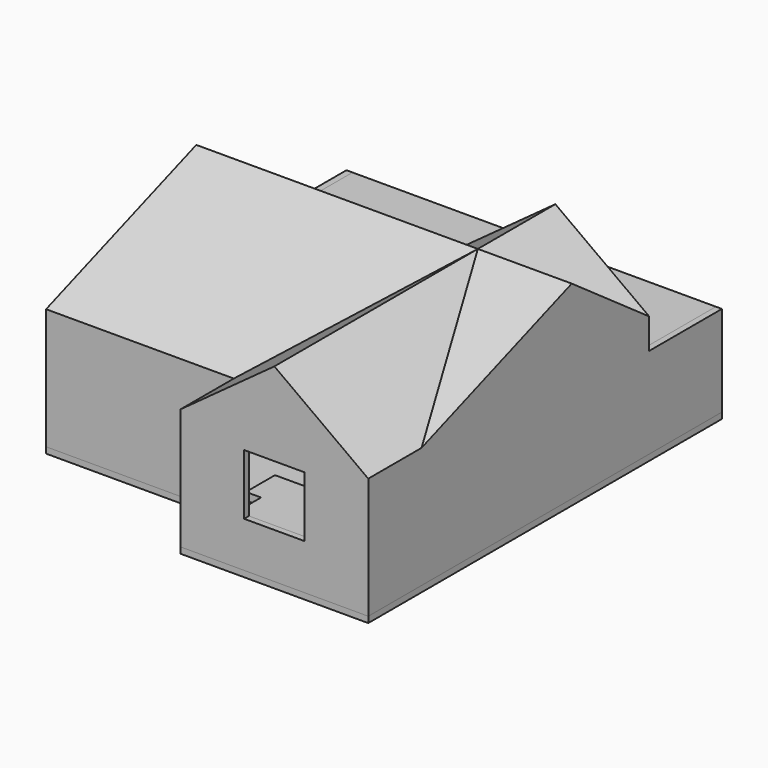
from build123d import *

# Parameters (mm, degrees)
F14_DEPTH    = 12400
F15_W        = 2000
F15_H        = 1000
F0_DEPTH     = 11600
F16_DEPTH    = 4000
F1_T         = 200
F1_T3_DEPTH  = 7689.8774544047
F1_T5_DEPTH  = 5394.2279984236
F1_T7_DEPTH  = 5394.2279984236
F1_T9_DEPTH  = 7689.8774544047
F1_T11_DEPTH = 4400
F2_W         = 2000
F2_H         = 2000
F17_DEPTH    = 2400
F18_DEPTH    = 200
F3_W         = 1000
F3_H         = 500
F3_W_2       = 500
F3_H_2       = 1000
F3_H_3       = 200
F4_DEPTH     = 200
F5_START     = -2800
F5_DEPTH     = 200
F6_START     = -1200
F6_DEPTH     = 300
F7_START     = -1450
F7_DEPTH     = 300
F19_START    = -1700
F19_DEPTH    = 300
F20_START    = -1950
F20_DEPTH    = 300
F21_START    = -2200
F21_DEPTH    = 300
F8_START     = -2450
F8_DEPTH     = 300
F22_START    = -2700
F22_DEPTH    = 300
F9_START     = -950
F9_DEPTH     = 300
F10_START    = -700
F10_DEPTH    = 300
F11_START    = -450
F11_DEPTH    = 300
F23_START    = -200
F23_DEPTH    = 300
F12_DEPTH    = 250


# Not quite as in the source:
# - an extrude ends at something that could not be found from the text; its depth is read off the source's solid
# - a shell that OpenCascade refuses in one call is made with other operations: the cavity is built on its own and cut out


with BuildPart() as f14:
    # F13 (on Right) → F14 (new body)
    with BuildSketch(Plane.YZ):
        Polygon((-6200, 0), (6200, 0), (6200, 3000), (3200, 3000), (3200, 4000), (0, 6256.6154524505), (-6200, 4000), align=None)
    extrude(amount=F14_DEPTH)

    # F15 (on face) → F0 (join)
    with BuildSketch(Plane(origin=(0, 3200, 0), x_dir=(-1, 0, 0), z_dir=(0, 1, 0))):
        Polygon((-9300, 6256.6154524505), (-12400, 4000), (-10300, 4000), (-10300, 5000), (-8300, 5000), (-8300, 4000), (-6200, 4000), align=None)
        with Locations((-9300, 4500)):
            Rectangle(F15_W, F15_H)
    extrude(amount=-F0_DEPTH)

    # F16 (add, through all): a face of the model
    f16_faces = [f14.faces().sort_by_distance(p)[0] for p in [
        (9300, -7300, 4000),
    ]]
    extrude(f16_faces, amount=F16_DEPTH)

    # F1: shell of thickness 200, made by hand


with BuildPart() as f1_core1:
    # F1_t2: copy of F14
    add(f14.part)

    # the walls: a layer under each face that stays
    f1_faces = [f1_core1.faces().sort_by_distance(p)[0] for p in [
        (4650, -3100, 5128.3077262252),
        (4650, 1600, 5128.3077262252),
        (10333.3333333333, 3200, 3542.7692420751),
        (9816.6666666667, 1600, 5880.512877042),
        (11883.3333333333, 1600, 5128.3077262252),
        (11883.3333333333, -1033.3333333333, 5880.512877042),
        (10850, -4200, 5128.3077262252),
        (9300, -8400, 3128.3077262252),
        (6200, -7300, 2000),
        (12400, -1100, 3128.3077262252),
        (7750, 2666.6666666667, 5128.3077262252),
        (7750, -4200, 5128.3077262252),
        (3100, -6200, 2000),
        (0, 0, 3128.3077262252),
    ]]
    thicken(f1_faces, amount=-F1_T, mode=Mode.SUBTRACT)

    # F1_s4 → F1_t3 (cut)
    with BuildSketch(Plane(origin=(-679.6785869535, -1359.357173907, -494.7655490384), x_dir=(-0.894427191, 0.4472135955, 0), z_dir=(0.4252472033, 0.8504944066, 0.3095546484))):
        Polygon((-8317.4260033625, 4665.513258174), (-8287.5816646932, 4464.1897106586), (-8360.6155438547, 4452.8857222652), (-8423.4513815758, 4491.7879735735), align=None)
    extrude(amount=F1_T3_DEPTH, mode=Mode.SUBTRACT)

    # F1_s6 → F1_t5 (cut)
    with BuildSketch(Plane(origin=(5462.1086087811, -5638.3056606773, 3976.089899851), x_dir=(-0.7182402228, -0.6957952158, 0), z_dir=(-0.6207165554, 0.6407396701, -0.4518447002))):
        Polygon((-6679.5906506398, 2661.3103147543), (-6599.4357743978, 2474.4492579485), (-6682.2486847174, 2438.2000137734), (-6764.1744994282, 2476.4118797687), align=None)
    extrude(amount=F1_T5_DEPTH, mode=Mode.SUBTRACT)

    # F1_s8 → F1_t7 (cut)
    with BuildSketch(Plane(origin=(5052.5541970253, 5215.5398162841, -3677.9586694679), x_dir=(0.7182402228, -0.6957952158, 0), z_dir=(-0.6207165554, -0.6407396701, 0.4518447002))):
        Polygon((6679.6774932388, 8508.9899951089), (6595.0936444505, 8324.0915601233), (6677.0194591612, 8285.8796941281), (6759.8323694808, 8322.1289383031), align=None)
    extrude(amount=F1_T7_DEPTH, mode=Mode.SUBTRACT)

    # F1_s10 → F1_t9 (cut)
    with BuildSketch(Plane(origin=(773.1141266852, -1546.2282533704, -562.7810596082), x_dir=(0.894427191, 0.4472135955, 0), z_dir=(0.4252472033, -0.8504944066, -0.3095546484))):
        Polygon((8318.9197492359, 7240.4423384247), (8348.7640879052, 7039.1187909094), (8275.7302087437, 7027.8148025159), (8212.8943710226, 7066.7170538243), align=None)
    extrude(amount=F1_T9_DEPTH, mode=Mode.SUBTRACT)

    # F1_s12 → F1_t11 (cut)
    with BuildSketch(Plane.XY.offset(-200)):
        Polygon((6198, -6202), (6400, -6200), (6400, -6000), (6200, -6000), align=None)
    extrude(amount=F1_T11_DEPTH, mode=Mode.SUBTRACT)


with BuildPart() as f14_1:
    add(f14.part)

    # what is left inside the walls is the cavity
    f1_cavity = [f1_core1.part.solids().sort_by_distance(p)[0] for p in [
        (8200, -1000, 2),
    ]]
    add(f1_cavity, mode=Mode.SUBTRACT)

    # F2 (on face) → F17 (cut, through all)
    with BuildSketch(Plane.XZ.offset(8400)):
        with Locations((9300, 2500)):
            Rectangle(F2_W, F2_H)
    extrude(amount=-F17_DEPTH, mode=Mode.SUBTRACT)

    # F15 (on face) → F18 (cut, through all)
    with BuildSketch(Plane(origin=(0, 3200, 0), x_dir=(-1, 0, 0), z_dir=(0, 1, 0))):
        with Locations((-9300, 3500)):
            Rectangle(F15_W, F15_H)
        with Locations((-9300, 4500)):
            Rectangle(F15_W, F15_H)
    extrude(amount=-F18_DEPTH, mode=Mode.SUBTRACT)


with BuildPart() as f4:
    # F3 (on face) → F4 (new body)
    with BuildSketch(Plane(origin=(0, 0, 0), x_dir=(1, 0, 0), z_dir=(0, 0, -1))):
        Polygon((200, 6000), (6400, 6000), (6400, 6200), (6400, 6700), (6400, 7200), (6400, 8200), (7400, 8200), (7900, 8200), (10700, 8200), (11200, 8200), (12200, 8200), (12200, 7200), (12200, 6700), (12200, 6200), (12200, 6000), (12200, -6200), (12400, -6200), (12400, 8400), (6200, 8400), (6200, 6200), (0, 6200), (0, -6200), (200, -6200), align=None)
        Polygon((7400, 6000), (6400, 6000), (200, 6000), (200, -6200), (12200, -6200), (12200, 6000), (11200, 6000), align=None)
        Polygon((6400, 8200), (6400, 7200), (7400, 7200), align=None)
        with Locations((6900, 6950)):
            Rectangle(F3_W, F3_H)
        Polygon((7400, 8200), (6400, 8200), (7400, 7200), align=None)
        with Locations((7650, 7700)):
            Rectangle(F3_W_2, F3_H_2)
        Polygon((7400, 6200), (7400, 6000), (11200, 6000), (11200, 6200), (11200, 6700), (11200, 7200), (10700, 7200), (10700, 8200), (7900, 8200), (7900, 7200), (7400, 7200), (7400, 6700), align=None)
        with Locations((6900, 6450)):
            Rectangle(F3_W, F3_H)
        with Locations((6900, 6100)):
            Rectangle(F3_W, F3_H_3)
        with Locations((11700, 6100)):
            Rectangle(F3_W, F3_H_3)
        with Locations((11700, 6450)):
            Rectangle(F3_W, F3_H)
        with Locations((11700, 6950)):
            Rectangle(F3_W, F3_H)
        Polygon((12200, 8200), (11200, 7200), (12200, 7200), align=None)
        Polygon((11200, 8200), (11200, 7200), (12200, 8200), align=None)
        with Locations((10950, 7700)):
            Rectangle(F3_W_2, F3_H_2)
    extrude(amount=F4_DEPTH)


with BuildPart() as f5:
    # F3 (on face) → F5 (new body)
    with BuildSketch(Plane(origin=(0, 0, 0), x_dir=(1, 0, 0), z_dir=(0, 0, -1)).offset(F5_START)):
        Polygon((7400, 6000), (6400, 6000), (200, 6000), (200, -6200), (12200, -6200), (12200, 6000), (11200, 6000), align=None)
    extrude(amount=-F5_DEPTH)


with BuildPart() as f6:
    # F3 (on face) → F6 (new body)
    with BuildSketch(Plane(origin=(0, 0, 0), x_dir=(1, 0, 0), z_dir=(0, 0, -1)).offset(F6_START)):
        Polygon((7400, 6200), (7400, 6000), (11200, 6000), (11200, 6200), (11200, 6700), (11200, 7200), (10700, 7200), (10700, 8200), (7900, 8200), (7900, 7200), (7400, 7200), (7400, 6700), align=None)
    extrude(amount=-F6_DEPTH)

    # F3 (on face) → F7 (join)
    with BuildSketch(Plane(origin=(0, 0, 0), x_dir=(1, 0, 0), z_dir=(0, 0, -1)).offset(F7_START)):
        with Locations((10950, 7700)):
            Rectangle(F3_W_2, F3_H_2)
    extrude(amount=-F7_DEPTH)

    # F3 (on face) → F19 (join)
    with BuildSketch(Plane(origin=(0, 0, 0), x_dir=(1, 0, 0), z_dir=(0, 0, -1)).offset(F19_START)):
        Polygon((11200, 8200), (11200, 7200), (12200, 8200), align=None)
    extrude(amount=-F19_DEPTH)

    # F3 (on face) → F20 (join)
    with BuildSketch(Plane(origin=(0, 0, 0), x_dir=(1, 0, 0), z_dir=(0, 0, -1)).offset(F20_START)):
        Polygon((12200, 8200), (11200, 7200), (12200, 7200), align=None)
    extrude(amount=-F20_DEPTH)

    # F3 (on face) → F21 (join)
    with BuildSketch(Plane(origin=(0, 0, 0), x_dir=(1, 0, 0), z_dir=(0, 0, -1)).offset(F21_START)):
        with Locations((11700, 6950)):
            Rectangle(F3_W, F3_H)
    extrude(amount=-F21_DEPTH)

    # F3 (on face) → F8 (join)
    with BuildSketch(Plane(origin=(0, 0, 0), x_dir=(1, 0, 0), z_dir=(0, 0, -1)).offset(F8_START)):
        with Locations((11700, 6450)):
            Rectangle(F3_W, F3_H)
    extrude(amount=-F8_DEPTH)

    # F3 (on face) → F22 (join)
    with BuildSketch(Plane(origin=(0, 0, 0), x_dir=(1, 0, 0), z_dir=(0, 0, -1)).offset(F22_START)):
        with Locations((11700, 6100)):
            Rectangle(F3_W, F3_H_3)
    extrude(amount=-F22_DEPTH)

    # F3 (on face) → F9 (join)
    with BuildSketch(Plane(origin=(0, 0, 0), x_dir=(1, 0, 0), z_dir=(0, 0, -1)).offset(F9_START)):
        with Locations((7650, 7700)):
            Rectangle(F3_W_2, F3_H_2)
    extrude(amount=-F9_DEPTH)

    # F3 (on face) → F10 (join)
    with BuildSketch(Plane(origin=(0, 0, 0), x_dir=(1, 0, 0), z_dir=(0, 0, -1)).offset(F10_START)):
        Polygon((7400, 8200), (6400, 8200), (7400, 7200), align=None)
    extrude(amount=-F10_DEPTH)

    # F3 (on face) → F11 (join)
    with BuildSketch(Plane(origin=(0, 0, 0), x_dir=(1, 0, 0), z_dir=(0, 0, -1)).offset(F11_START)):
        Polygon((6400, 8200), (6400, 7200), (7400, 7200), align=None)
    extrude(amount=-F11_DEPTH)

    # F3 (on face) → F23 (join)
    with BuildSketch(Plane(origin=(0, 0, 0), x_dir=(1, 0, 0), z_dir=(0, 0, -1)).offset(F23_START)):
        with Locations((6900, 6950)):
            Rectangle(F3_W, F3_H)
    extrude(amount=-F23_DEPTH)

    # F3 (on face) → F12 (join)
    with BuildSketch(Plane(origin=(0, 0, 0), x_dir=(1, 0, 0), z_dir=(0, 0, -1))):
        with Locations((6900, 6450)):
            Rectangle(F3_W, F3_H)
    extrude(amount=-F12_DEPTH)


solid = Compound([f14_1.part, f4.part, f5.part, f6.part])
